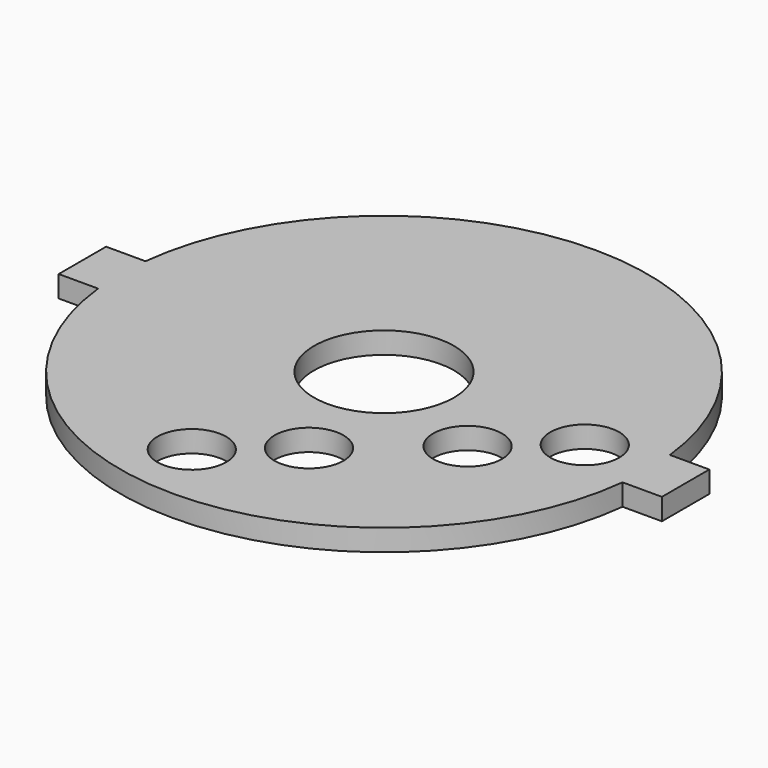
from build123d import *

# Parameters (mm, degrees)
F0_R     = 3.2
F0_R_2   = 6.5
F1_DEPTH = 2


# Not quite as in the source:
# - a feature names something its author has since deleted; it is built from what else it names


with BuildPart() as f1:
    # F0 (on Top) → F1 (new body)
    with BuildSketch(Plane.XY):
        with BuildLine():
            Line((21, 2.75), (24.3451740598, 2.75))
            ThreePointArc((24.3451740598, 2.75), (0, 24.5), (-24.3451740598, 2.75))
            Line((-24.3451740598, 2.75), (-21, 2.75))
            Line((-21, 2.75), (-21, -2.75))
            Line((-21, -2.75), (-24.3451740598, -2.75))
            ThreePointArc((-24.3451740598, -2.75), (0, -24.5), (24.3451740598, -2.75))
            Line((24.3451740598, -2.75), (21, -2.75))
            Line((21, -2.75), (21, -1.9091370521))
            ThreePointArc((21, -1.9091370521), (15.3353042136, 0.1317634061), (21, 2.1726638643))
            Line((21, 2.1726638643), (21, 2.75))
        make_face()
        with Locations((-3.267275868, -18.2230044156)):
            Circle(F0_R, mode=Mode.SUBTRACT)
        with Locations((3.235248016, -12.7487754162)):
            Circle(F0_R, mode=Mode.SUBTRACT)
        Circle(F0_R_2, mode=Mode.SUBTRACT)
        with Locations((12.0327803296, -5.3424655934)):
            Circle(F0_R, mode=Mode.SUBTRACT)
        with BuildLine():
            Line((-21, 2.75), (-24.3451740598, 2.75))
            ThreePointArc((-24.3451740598, 2.75), (-24.5, 0), (-24.3451740598, -2.75))
            Line((-24.3451740598, -2.75), (-21, -2.75))
            Line((-21, -2.75), (-21, 2.75))
        make_face()
        with BuildLine():
            ThreePointArc((-24.3451740598, -2.75), (-24.5, 0), (-24.3451740598, 2.75))
            Line((-24.3451740598, 2.75), (-28, 2.75))
            Line((-28, 2.75), (-28, -2.75))
            Line((-28, -2.75), (-24.3451740598, -2.75))
        make_face()
        with BuildLine():
            ThreePointArc((24.3451740598, -2.75), (24.4612628912, -1.3771774642), (24.5, 0))
            ThreePointArc((24.5, 0), (24.4612628912, 1.3771774642), (24.3451740598, 2.75))
            Line((24.3451740598, 2.75), (21, 2.75))
            Line((21, 2.75), (21, 2.1726638643))
            ThreePointArc((21, 2.1726638643), (21.5458711466, 1.2164231415), (21.7353042136, 0.1317634061))
            ThreePointArc((21.7353042136, 0.1317634061), (21.5458711466, -0.9528963294), (21, -1.9091370521))
            Line((21, -1.9091370521), (21, -2.75))
            Line((21, -2.75), (24.3451740598, -2.75))
        make_face()
        with BuildLine():
            ThreePointArc((24.3451740598, 2.75), (24.4612628912, 1.3771774642), (24.5, 0))
            ThreePointArc((24.5, 0), (24.4612628912, -1.3771774642), (24.3451740598, -2.75))
            Line((24.3451740598, -2.75), (28, -2.75))
            Line((28, -2.75), (28, 2.75))
            Line((28, 2.75), (24.3451740598, 2.75))
        make_face()
    extrude(amount=F1_DEPTH)


solid = f1.part
